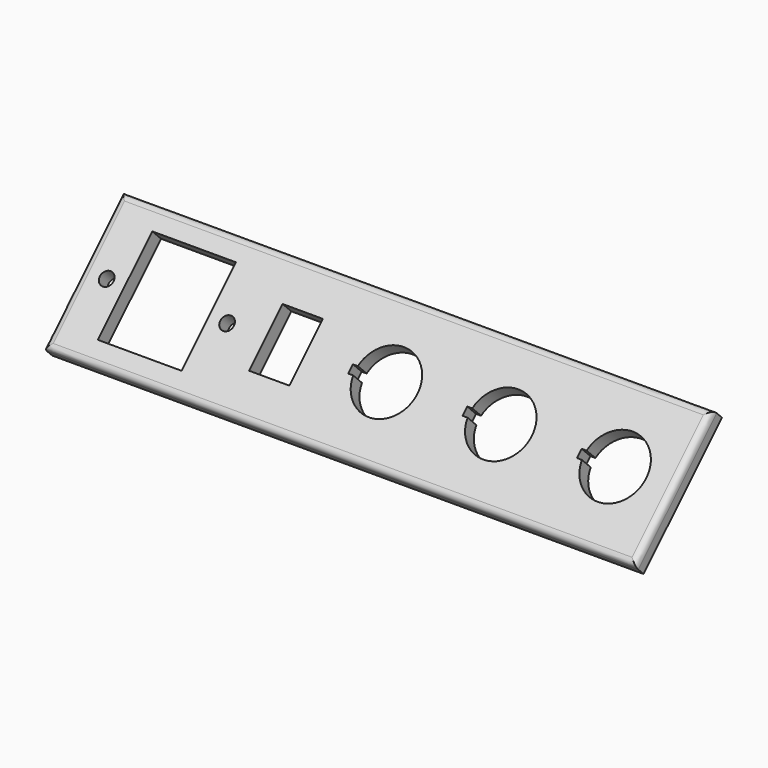
from build123d import *

# Parameters (mm, degrees)
F0_W        = 190
F0_H        = 44.5
F1_DEPTH    = 5
F2_W        = 26.885152871
F2_H        = 30.8681384815
F2_W_2      = 12.9447032342
F2_H_2      = 19
F3_DEPTH    = 5.001
F4_D        = 4.4
F5_ANGLE    = -45
F6_T1_DEPTH = 54.5
F6_T3_DEPTH = 200
F6_T5_DEPTH = 54.5


# Not quite as in the source:
# - a fillet or chamfer that OpenCascade refuses, or shapes differently, is made with other operations: its cross-section is extruded or revolved along the edge and cut away or added


with BuildPart() as f1:
    # F0 (on Top) → F1 (new body)
    with BuildSketch(Plane.XY):
        Rectangle(F0_W, F0_H)
    extrude(amount=F1_DEPTH)

    # F2 (on face) → F3 (cut, through all)
    with BuildSketch(Plane.XY.offset(5)):
        with Locations((-67.9330339405, 0)):
            Rectangle(F2_W, F2_H)
        with Locations((-29.686499387, 0.061675)):
            Rectangle(F2_W_2, F2_H_2)
        with BuildLine():
            Line((-8.9000007138, -1.3249999611), (-7.3118307668, -1.3249999611))
            ThreePointArc((-7.3118307668, -1.3249999611), (12.5999992862, 3.89e-08), (-7.3118307668, 1.3250000389))
            Line((-7.3118307668, 1.3250000389), (-8.9000007138, 1.3250000389))
            Line((-8.9000007138, 1.3250000389), (-8.9000007138, -1.3249999611))
        make_face()
        with BuildLine():
            Line((27.8544989455, -1.3249999611), (29.4426688924, -1.3249999611))
            ThreePointArc((29.4426688924, -1.3249999611), (49.3544989455, 3.89e-08), (29.4426688924, 1.3250000389))
            Line((29.4426688924, 1.3250000389), (27.8544989455, 1.3250000389))
            Line((27.8544989455, 1.3250000389), (27.8544989455, -1.3249999611))
        make_face()
        with BuildLine():
            Line((64.6044989455, -1.3293345302), (66.1926688924, -1.3293345302))
            ThreePointArc((66.1926688924, -1.3293345302), (86.1044989455, -0.0043345302), (66.1926688924, 1.3206654698))
            Line((66.1926688924, 1.3206654698), (64.6044989455, 1.3206654698))
            Line((64.6044989455, 1.3206654698), (64.6044989455, -1.3293345302))
        make_face()
    extrude(amount=-F3_DEPTH, mode=Mode.SUBTRACT)

    # F4 (through all)
    with Locations(Plane.XY.offset(5)):
        with Locations((-87.275610376, 0), (-48.590457505, 0)):
            Hole(F4_D / 2)


with BuildPart() as f1_1:
    # F5: moved
    add(f1.part.rotate(Axis((0, -22.25, 5), (-1, 0, 0)), F5_ANGLE))

    # F6: fillet of radius 2 on 4 edges, made by hand

    # F6_s2 → F6_t1 (cut)
    with BuildSketch(Plane(origin=(0, 26.3767856687, 26.3767856687), x_dir=(1, 0, 0), z_dir=(0, -0.7071067812, -0.7071067812))):
        with BuildLine():
            add(Edge.make_bspline(
                [(-95, 17.2686597873), (-95, 19.2686597873), (-93, 19.2686597873)],
                knots=[0, 0, 0, 1, 1, 1], degree=2, weights=[1, 1, 1]))
            Line((-93, 19.2686597873), (-95, 19.2686597873))
            Line((-95, 19.2686597873), (-95, 17.2686597873))
        make_face()
    extrude(amount=F6_T1_DEPTH, mode=Mode.SUBTRACT)

    # F6_s4 → F6_t3 (cut)
    with BuildSketch(Plane.YZ.offset(-100)):
        with BuildLine():
            add(Edge.make_bspline(
                [(7.8020382004, 35.0520382004), (9.2162517628, 36.4662517628), (10.6304653252, 35.0520382004)],
                knots=[0, 0, 0, 1, 1, 1], degree=2, weights=[1, 1, 1]))
            Line((10.6304653252, 35.0520382004), (9.2162517628, 36.4662517628))
            Line((9.2162517628, 36.4662517628), (7.8020382004, 35.0520382004))
        make_face()
        with BuildLine():
            add(Edge.make_bspline(
                [(-20.8357864376, 3.5857864376), (-22.25, 5), (-20.8357864376, 6.4142135624)],
                knots=[0, 0, 0, 1, 1, 1], degree=2, weights=[1, 1, 1]))
            Line((-20.8357864376, 6.4142135624), (-22.25, 5))
            Line((-22.25, 5), (-20.8357864376, 3.5857864376))
        make_face()
    extrude(amount=F6_T3_DEPTH, mode=Mode.SUBTRACT)

    # F6_s6 → F6_t5 (cut)
    with BuildSketch(Plane(origin=(0, -12.1605339059, -12.1605339059), x_dir=(1, 0, 0), z_dir=(0, 0.7071067812, 0.7071067812))):
        with BuildLine():
            add(Edge.make_bspline(
                [(95, -17.2686597873), (95, -19.2686597873), (93, -19.2686597873)],
                knots=[0, 0, 0, 1, 1, 1], degree=2, weights=[1, 1, 1]))
            Line((93, -19.2686597873), (95, -19.2686597873))
            Line((95, -19.2686597873), (95, -17.2686597873))
        make_face()
    extrude(amount=F6_T5_DEPTH, mode=Mode.SUBTRACT)


solid = f1_1.part
